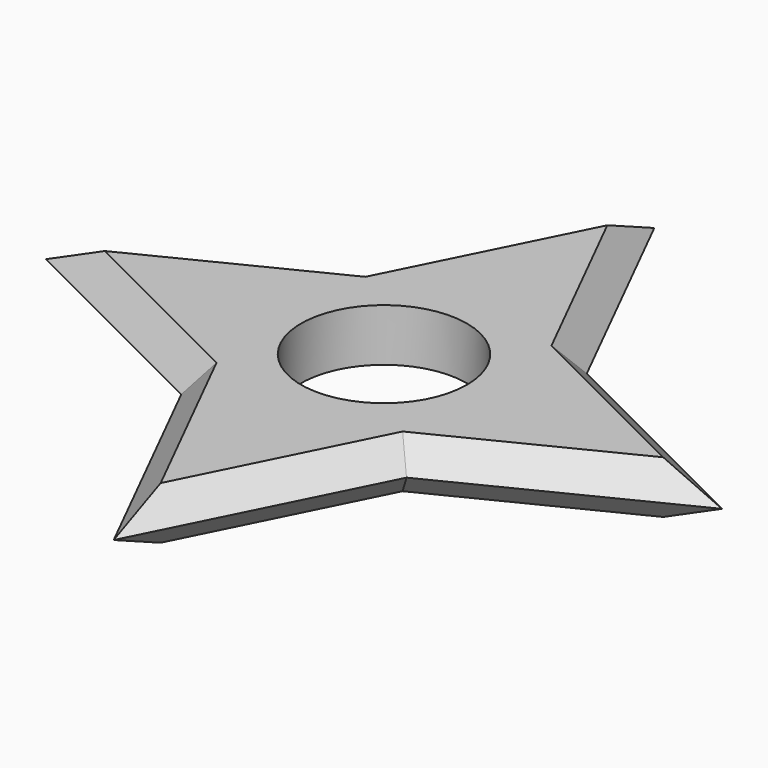
from build123d import *

# Parameters (mm, degrees)
F0_R     = 11.05
F1_DEPTH = 7
F2_SIZE  = 3.5
F3_SIZE  = 3.49999


# Not quite as in the source:
# - a fillet or chamfer is up to 0.001 mm smaller than in the source, because OpenCascade refuses the exact size


with BuildPart() as f1:
    # F0 (on Top) → F1 (new body)
    with BuildSketch(Plane.XY):
        Polygon((0, 45), (-15, 15), (0, 15), align=None)
        Polygon((0, 45), (0, 15), (15, 15), align=None)
        Polygon((0, 15), (-15, 15), (-15, 0), (-15, -15), (0, -15), (15, -15), (15, 0), (15, 15), align=None)
        Circle(F0_R, mode=Mode.SUBTRACT)
        Polygon((-15, -15), (-15, 0), (-45, 0), align=None)
        Polygon((-15, 0), (-15, 15), (-45, 0), align=None)
        Polygon((0, -15), (-15, -15), (0, -45), align=None)
        Polygon((15, -15), (0, -15), (0, -45), align=None)
        Polygon((45, 0), (15, 0), (15, -15), align=None)
        Polygon((45, 0), (15, 15), (15, 0), align=None)
    extrude(amount=F1_DEPTH)

    # F2
    f2_edges = [f1.edges().sort_by_distance(p)[0] for p in [
        (30, -7.5, 7),
        (7.5, -30, 7),
        (-7.5, -30, 7),
        (-30, -7.5, 7),
        (-30, 7.5, 7),
        (-7.5, 30, 7),
        (7.5, 30, 7),
        (30, 7.5, 7),
    ]]
    chamfer(f2_edges, length=F2_SIZE)

    # F3 (size 3.5 in the source; OpenCascade refuses exactly that, so slightly less here)
    f3_edges = [f1.edges().sort_by_distance(p)[0] for p in [
        (30, 7.5, 0),
        (7.5, 30, 0),
        (-7.5, 30, 0),
        (-30, 7.5, 0),
        (-30, -7.5, 0),
        (-7.5, -30, 0),
        (7.5, -30, 0),
        (30, -7.5, 0),
    ]]
    chamfer(f3_edges, length=F3_SIZE)


solid = f1.part
